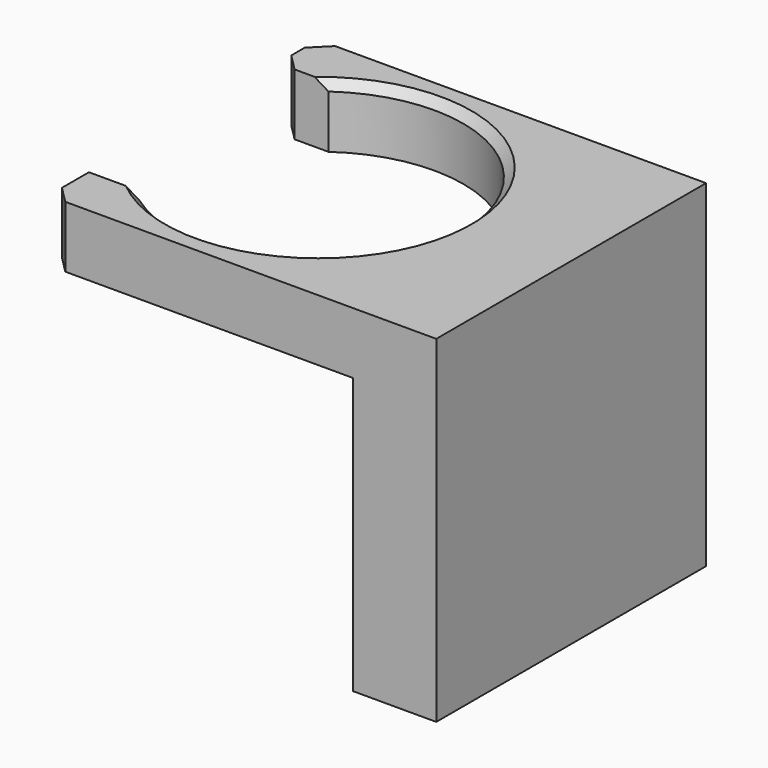
from build123d import *

# Parameters (mm, degrees)
F1_DEPTH = 3.65
F2_SIZE  = 1
F3_SIZE  = 0.5
F4_W     = 4.925
F4_H     = 20
F5_DEPTH = 20


with BuildPart() as f1:
    # F0 (on Top) → F1 (new body)
    with BuildSketch(Plane.XY):
        with BuildLine():
            ThreePointArc((-4.9959983987, 7), (8.6, 0), (-4.9959983987, -7))
            Line((-4.9959983987, -7), (-8, -7))
            Line((-8, -7), (-8, -10))
            Line((-8, -10), (8, -10))
            Line((8, -10), (15, -10))
            Line((15, -10), (15, 10))
            Line((15, 10), (8, 10))
            Line((8, 10), (-8, 10))
            Line((-8, 10), (-8, 7))
            Line((-8, 7), (-4.9959983987, 7))
        make_face()
    extrude(amount=F1_DEPTH)

    # F2
    f2_edges = [f1.edges().sort_by_distance(p)[0] for p in [
        (-8, 10, 1.825),
        (-8, 7, 1.825),
        (-8, -10, 1.825),
    ]]
    chamfer(f2_edges, length=F2_SIZE)

    # F3
    f3_edges = [f1.edges().sort_by_distance(p)[0] for p in [
        (8.6, 0, 3.65),
    ]]
    chamfer(f3_edges, length=F3_SIZE)

    # F4 (on face) → F5 (join)
    with BuildSketch(Plane.XY.offset(3.65)):
        with Locations((12.5375, 0)):
            Rectangle(F4_W, F4_H)
    extrude(amount=-F5_DEPTH)


solid = f1.part
